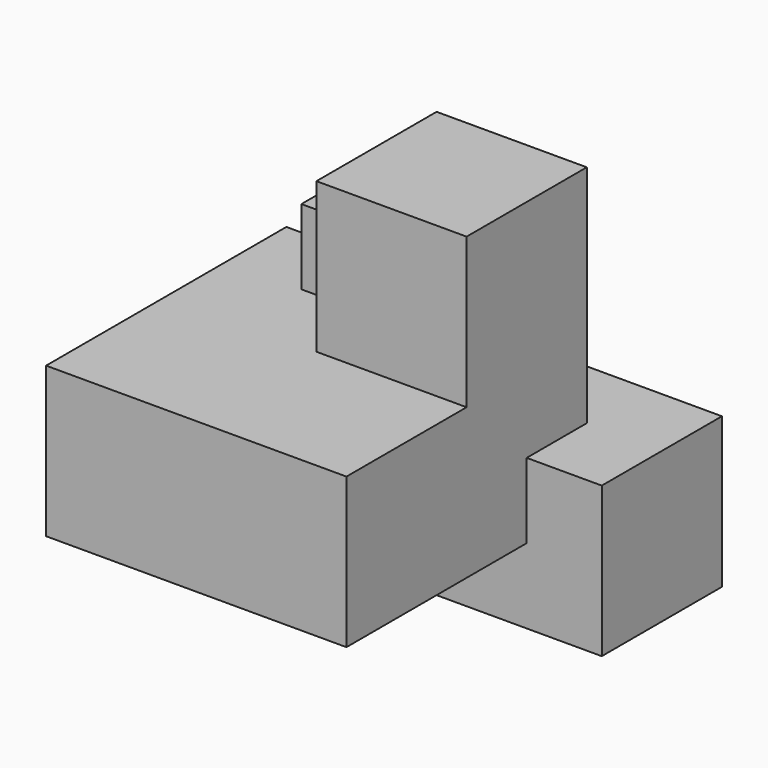
from build123d import *

# Parameters (mm, degrees)
F0_W     = 19.05
F0_H     = 19.05
F1_DEPTH = 9.525
F2_W     = 19.05
F2_H     = 19.05
F3_DEPTH = 38.1
F4_DEPTH = 19.05


with BuildPart() as f1:
    # F0 (on Front) → F1 (new body, symmetric)
    with BuildSketch(Plane.XZ):
        Rectangle(F0_W, F0_H)
        with Locations((-19.05, -19.05)):
            Rectangle(F0_W, F0_H)
        with Locations((0, -19.05)):
            Rectangle(F0_W, F0_H)
        with Locations((19.05, -19.05)):
            Rectangle(F0_W, F0_H)
    extrude(amount=F1_DEPTH, both=True)


with BuildPart() as f3:
    # F2 (on Front) → F3 (new body)
    with BuildSketch(Plane.XZ):
        with Locations((-9.525, -9.525)):
            Rectangle(F2_W, F2_H)
        with Locations((9.525, -9.525)):
            Rectangle(F2_W, F2_H)
    extrude(amount=F3_DEPTH)

    # F2 (on Front) → F4 (join)
    with BuildSketch(Plane.XZ):
        with Locations((-9.525, -9.525)):
            Rectangle(F2_W, F2_H)
        with Locations((9.525, -9.525)):
            Rectangle(F2_W, F2_H)
        with Locations((9.525, 9.525)):
            Rectangle(F2_W, F2_H)
    extrude(amount=F4_DEPTH)


solid = Compound([f1.part, f3.part])
